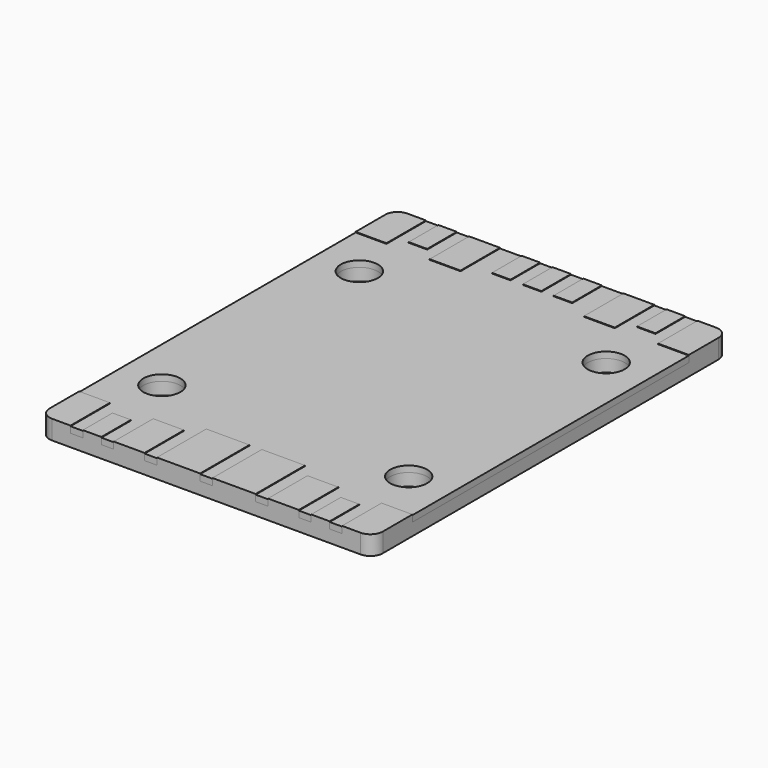
from build123d import *

# Parameters (mm, degrees)
F0_R     = 1.5
F0_W     = 1.5
F0_H     = 3
F0_W_2   = 2.5
F0_H_2   = 4
F0_W_3   = 3.5
F0_H_3   = 5
F1_DEPTH = 1.5
F2_DEPTH = 1
F3_DEPTH = 1.55


# Not quite as in the source:
# - a feature names something its author has since deleted; it is built from what else it names


with BuildPart() as f1:
    # F0 (on Top) → F1 (new body)
    with BuildSketch(Plane.XY):
        with BuildLine():
            ThreePointArc((13.5, 17), (13.2071067812, 17.7071067812), (12.5, 18))
            Line((12.5, 18), (11, 18))
            Line((11, 18), (11, 14))
            Line((11, 14), (13.5, 14))
            Line((13.5, 14), (13.5, 17))
        make_face()
        Polygon((11, 14), (11, 18), (10, 18), (10, 15), (8.5, 15), (8.5, 18), (7.5, 18), (7.5, 14), (5, 14), (5, 18), (3.25, 18), (3.25, 15), (1.75, 15), (1.75, 18), (0.75, 18), (0.75, 15), (-0.75, 15), (-0.75, 18), (-1.75, 18), (-1.75, 15), (-3.25, 15), (-3.25, 18), (-5, 18), (-5, 14), (-7.5, 14), (-7.5, 18), (-8.5, 18), (-8.5, 15), (-10, 15), (-10, 18), (-11, 18), (-11, 14), (-13.5, 14), (-13.5, -14), (-11, -14), (-11, -18), (-10, -18), (-10, -15), (-8.5, -15), (-8.5, -18), (-7.5, -18), (-7.5, -14), (-5, -14), (-5, -18), (-4, -18), (-4, -13), (-0.5, -13), (-0.5, -18), (0.5, -18), (0.5, -13), (4, -13), (4, -18), (5, -18), (5, -14), (7.5, -14), (7.5, -18), (8.5, -18), (8.5, -15), (10, -15), (10, -18), (11, -18), (11, -14), (13.5, -14), (13.5, 14), align=None)
        with Locations((-10, -10)):
            Circle(F0_R, mode=Mode.SUBTRACT)
        with Locations((10, -10)):
            Circle(F0_R, mode=Mode.SUBTRACT)
        with Locations((-10, 10)):
            Circle(F0_R, mode=Mode.SUBTRACT)
        with Locations((10, 10)):
            Circle(F0_R, mode=Mode.SUBTRACT)
        with Locations((9.25, 16.5)):
            Rectangle(F0_W, F0_H)
        with BuildLine():
            Line((13.5, -17), (13.5, -14))
            Line((13.5, -14), (11, -14))
            Line((11, -14), (11, -18))
            Line((11, -18), (12.5, -18))
            ThreePointArc((12.5, -18), (13.2071067812, -17.7071067812), (13.5, -17))
        make_face()
        with Locations((6.25, 16)):
            Rectangle(F0_W_2, F0_H_2)
        with Locations((2.5, 16.5)):
            Rectangle(F0_W, F0_H)
        with Locations((9.25, -16.5)):
            Rectangle(F0_W, F0_H)
        with Locations((0, 16.5)):
            Rectangle(F0_W, F0_H)
        with Locations((6.25, -16)):
            Rectangle(F0_W_2, F0_H_2)
        with Locations((-2.5, 16.5)):
            Rectangle(F0_W, F0_H)
        with Locations((2.25, -15.5)):
            Rectangle(F0_W_3, F0_H_3)
        with Locations((-6.25, 16)):
            Rectangle(F0_W_2, F0_H_2)
        with Locations((-2.25, -15.5)):
            Rectangle(F0_W_3, F0_H_3)
        with Locations((-9.25, 16.5)):
            Rectangle(F0_W, F0_H)
        with Locations((-6.25, -16)):
            Rectangle(F0_W_2, F0_H_2)
        with BuildLine():
            Line((-11, 14), (-11, 18))
            Line((-11, 18), (-12.5, 18))
            ThreePointArc((-12.5, 18), (-13.2071067812, 17.7071067812), (-13.5, 17))
            Line((-13.5, 17), (-13.5, 14))
            Line((-13.5, 14), (-11, 14))
        make_face()
        with Locations((-9.25, -16.5)):
            Rectangle(F0_W, F0_H)
        with BuildLine():
            Line((-12.5, -18), (-11, -18))
            Line((-11, -18), (-11, -14))
            Line((-11, -14), (-13.5, -14))
            Line((-13.5, -14), (-13.5, -17))
            ThreePointArc((-13.5, -17), (-13.2071067812, -17.7071067812), (-12.5, -18))
        make_face()
    extrude(amount=F1_DEPTH)


with BuildPart() as f2:
    # F0 (on Top) → F2 (new body)
    with BuildSketch(Plane.XY):
        with BuildLine():
            ThreePointArc((13.5, 17), (13.2071067812, 17.7071067812), (12.5, 18))
            Line((12.5, 18), (11, 18))
            Line((11, 18), (11, 14))
            Line((11, 14), (13.5, 14))
            Line((13.5, 14), (13.5, 17))
        make_face()
        Polygon((11, 14), (11, 18), (10, 18), (10, 15), (8.5, 15), (8.5, 18), (7.5, 18), (7.5, 14), (5, 14), (5, 18), (3.25, 18), (3.25, 15), (1.75, 15), (1.75, 18), (0.75, 18), (0.75, 15), (-0.75, 15), (-0.75, 18), (-1.75, 18), (-1.75, 15), (-3.25, 15), (-3.25, 18), (-5, 18), (-5, 14), (-7.5, 14), (-7.5, 18), (-8.5, 18), (-8.5, 15), (-10, 15), (-10, 18), (-11, 18), (-11, 14), (-13.5, 14), (-13.5, -14), (-11, -14), (-11, -18), (-10, -18), (-10, -15), (-8.5, -15), (-8.5, -18), (-7.5, -18), (-7.5, -14), (-5, -14), (-5, -18), (-4, -18), (-4, -13), (-0.5, -13), (-0.5, -18), (0.5, -18), (0.5, -13), (4, -13), (4, -18), (5, -18), (5, -14), (7.5, -14), (7.5, -18), (8.5, -18), (8.5, -15), (10, -15), (10, -18), (11, -18), (11, -14), (13.5, -14), (13.5, 14), align=None)
        with Locations((-10, -10)):
            Circle(F0_R, mode=Mode.SUBTRACT)
        with Locations((10, -10)):
            Circle(F0_R, mode=Mode.SUBTRACT)
        with Locations((-10, 10)):
            Circle(F0_R, mode=Mode.SUBTRACT)
        with Locations((10, 10)):
            Circle(F0_R, mode=Mode.SUBTRACT)
        with Locations((9.25, 16.5)):
            Rectangle(F0_W, F0_H)
        with BuildLine():
            Line((13.5, -17), (13.5, -14))
            Line((13.5, -14), (11, -14))
            Line((11, -14), (11, -18))
            Line((11, -18), (12.5, -18))
            ThreePointArc((12.5, -18), (13.2071067812, -17.7071067812), (13.5, -17))
        make_face()
        with Locations((6.25, 16)):
            Rectangle(F0_W_2, F0_H_2)
        with Locations((2.5, 16.5)):
            Rectangle(F0_W, F0_H)
        with Locations((9.25, -16.5)):
            Rectangle(F0_W, F0_H)
        with Locations((0, 16.5)):
            Rectangle(F0_W, F0_H)
        with Locations((6.25, -16)):
            Rectangle(F0_W_2, F0_H_2)
        with Locations((-2.5, 16.5)):
            Rectangle(F0_W, F0_H)
        with Locations((2.25, -15.5)):
            Rectangle(F0_W_3, F0_H_3)
        with Locations((-6.25, 16)):
            Rectangle(F0_W_2, F0_H_2)
        with Locations((-2.25, -15.5)):
            Rectangle(F0_W_3, F0_H_3)
        with Locations((-9.25, 16.5)):
            Rectangle(F0_W, F0_H)
        with Locations((-6.25, -16)):
            Rectangle(F0_W_2, F0_H_2)
        with BuildLine():
            Line((-11, 14), (-11, 18))
            Line((-11, 18), (-12.5, 18))
            ThreePointArc((-12.5, 18), (-13.2071067812, 17.7071067812), (-13.5, 17))
            Line((-13.5, 17), (-13.5, 14))
            Line((-13.5, 14), (-11, 14))
        make_face()
        with Locations((-9.25, -16.5)):
            Rectangle(F0_W, F0_H)
        with BuildLine():
            Line((-12.5, -18), (-11, -18))
            Line((-11, -18), (-11, -14))
            Line((-11, -14), (-13.5, -14))
            Line((-13.5, -14), (-13.5, -17))
            ThreePointArc((-13.5, -17), (-13.2071067812, -17.7071067812), (-12.5, -18))
        make_face()
    extrude(amount=F2_DEPTH)

    # F0 (on Top) → F3 (join)
    with BuildSketch(Plane.XY):
        with BuildLine():
            Line((-12.5, -18), (-11, -18))
            Line((-11, -18), (-11, -14))
            Line((-11, -14), (-13.5, -14))
            Line((-13.5, -14), (-13.5, -17))
            ThreePointArc((-13.5, -17), (-13.2071067812, -17.7071067812), (-12.5, -18))
        make_face()
        with Locations((-9.25, -16.5)):
            Rectangle(F0_W, F0_H)
        with Locations((-6.25, -16)):
            Rectangle(F0_W_2, F0_H_2)
        with Locations((-2.25, -15.5)):
            Rectangle(F0_W_3, F0_H_3)
        with Locations((2.25, -15.5)):
            Rectangle(F0_W_3, F0_H_3)
        with Locations((6.25, -16)):
            Rectangle(F0_W_2, F0_H_2)
        with Locations((9.25, -16.5)):
            Rectangle(F0_W, F0_H)
        with BuildLine():
            ThreePointArc((13.5, 17), (13.2071067812, 17.7071067812), (12.5, 18))
            Line((12.5, 18), (11, 18))
            Line((11, 18), (11, 14))
            Line((11, 14), (13.5, 14))
            Line((13.5, 14), (13.5, 17))
        make_face()
        with Locations((9.25, 16.5)):
            Rectangle(F0_W, F0_H)
        with Locations((6.25, 16)):
            Rectangle(F0_W_2, F0_H_2)
        with Locations((2.5, 16.5)):
            Rectangle(F0_W, F0_H)
        with Locations((0, 16.5)):
            Rectangle(F0_W, F0_H)
        with Locations((-2.5, 16.5)):
            Rectangle(F0_W, F0_H)
        with Locations((-6.25, 16)):
            Rectangle(F0_W_2, F0_H_2)
        with Locations((-9.25, 16.5)):
            Rectangle(F0_W, F0_H)
        with BuildLine():
            Line((-11, 14), (-11, 18))
            Line((-11, 18), (-12.5, 18))
            ThreePointArc((-12.5, 18), (-13.2071067812, 17.7071067812), (-13.5, 17))
            Line((-13.5, 17), (-13.5, 14))
            Line((-13.5, 14), (-11, 14))
        make_face()
        with BuildLine():
            Line((13.5, -17), (13.5, -14))
            Line((13.5, -14), (11, -14))
            Line((11, -14), (11, -18))
            Line((11, -18), (12.5, -18))
            ThreePointArc((12.5, -18), (13.2071067812, -17.7071067812), (13.5, -17))
        make_face()
    extrude(amount=F3_DEPTH)


solid = Compound([f1.part, f2.part])
